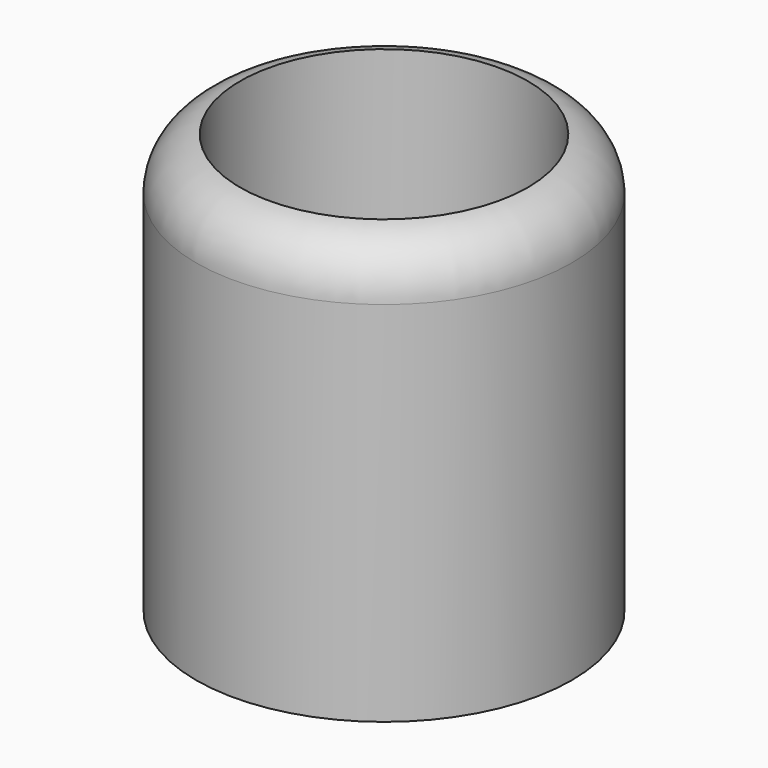
from build123d import *

# Parameters (mm, degrees)
F0_R     = 54.3589736978
F1_DEPTH = 121.412
F2_T     = -12.7


# Not quite as in the source:
# - a fillet or chamfer that OpenCascade refuses, or shapes differently, is made with other operations: its cross-section is extruded or revolved along the edge and cut away or added


with BuildPart() as f1:
    # F0 (on Top) → F1 (new body)
    with BuildSketch(Plane.XY):
        Circle(F0_R)
    extrude(amount=F1_DEPTH)

    # F2
    f2_openings = [f1.faces().sort_by_distance(p)[0] for p in [
        (0, 0, 121.412),
    ]]
    offset(amount=F2_T, openings=f2_openings)

    # F3: fillet of radius 15.3302561211 on 1 edges, made by hand

    # F3_s1 → F3_t2 (revolve, cut)
    with BuildSketch(Plane.XZ):
        with BuildLine():
            ThreePointArc((54.3589736978, 106.3090696395), (50.7619876396, 116.1755343746), (41.6589736978, 121.412))
            Line((41.6589736978, 121.412), (54.3589736978, 121.412))
            Line((54.3589736978, 121.412), (54.3589736978, 106.3090696395))
        make_face()
    revolve(axis=Axis((0, 0, 121.412), (0, 0, 1)), mode=Mode.SUBTRACT)


solid = f1.part
